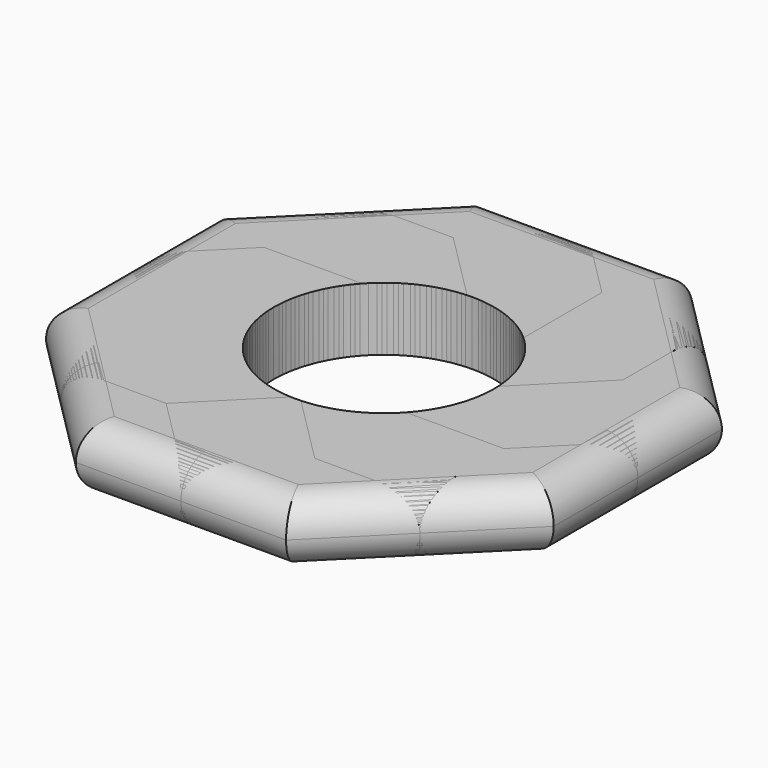
from build123d import *

# Parameters (mm, degrees)
F1_DEPTH = 3.175
F2_COUNT = 8
F3_R     = 11.049
F4_DEPTH = 12.7
F5_R     = 3.17499
F5_2_R   = 3.17499
F5_3_R   = 3.17499
F5_4_R   = 3.17499
F5_5_R   = 3.17499
F5_6_R   = 3.17499
F5_7_R   = 3.17499
F5_8_R   = 3.17499


# Not quite as in the source:
# - a fillet or chamfer is up to 0.001 mm smaller than in the source, because OpenCascade refuses the exact size


with BuildPart() as f1:
    # F0 (on Top) → F1 (new body, symmetric)
    with BuildSketch(Plane.XY):
        Polygon((5.2605122421, 0), (-5.2605122421, 0), (-12.7, -7.4394877579), (-12.7, -17.9605122421), (-5.2605122421, -25.4), (5.2605122421, -25.4), (12.7, -17.9605122421), (12.7, -7.4394877579), align=None)
    extrude(amount=F1_DEPTH, both=True)


with BuildPart() as f2_1:
    # F2: instance of F1
    add(f1.part.rotate(Axis((5.2605122421, 0, 0), (0, 0, 1)), 1 * 360 / F2_COUNT))


with BuildPart() as f2_2:
    # F2: instance of F1
    add(f1.part.rotate(Axis((5.2605122421, 0, 0), (0, 0, 1)), 2 * 360 / F2_COUNT))


with BuildPart() as f2_3:
    # F2: instance of F1
    add(f1.part.rotate(Axis((5.2605122421, 0, 0), (0, 0, 1)), 3 * 360 / F2_COUNT))


with BuildPart() as f2_4:
    # F2: instance of F1
    add(f1.part.rotate(Axis((5.2605122421, 0, 0), (0, 0, 1)), 4 * 360 / F2_COUNT))


with BuildPart() as f2_5:
    # F2: instance of F1
    add(f1.part.rotate(Axis((5.2605122421, 0, 0), (0, 0, 1)), 5 * 360 / F2_COUNT))


with BuildPart() as f2_6:
    # F2: instance of F1
    add(f1.part.rotate(Axis((5.2605122421, 0, 0), (0, 0, 1)), 6 * 360 / F2_COUNT))


with BuildPart() as f2_7:
    # F2: instance of F1
    add(f1.part.rotate(Axis((5.2605122421, 0, 0), (0, 0, 1)), 7 * 360 / F2_COUNT))


with BuildPart() as f4_tool:
    # F3 (on Top) → F4 (new body, symmetric)
    with BuildSketch(Plane.XY):
        with Locations((5.2605122421, 0)):
            Circle(F3_R)
    extrude(amount=F4_DEPTH, both=True)


with BuildPart() as f1_1:
    add(f1.part)

    # F4: cut by f4_tool
    add(f4_tool.part, mode=Mode.SUBTRACT)

    # F5#7 (radius 3.175 in the source; OpenCascade refuses exactly that, so slightly less here)
    f5_7_edges = [f1_1.edges().sort_by_distance(p)[0] for p in [
        (-8.980256, -21.680256, 3.175),
        (0, -25.4, 3.175),
        (-8.980256, -21.680256, -3.175),
        (0, -25.4, -3.175),
    ]]
    fillet(f5_7_edges, radius=F5_7_R)


with BuildPart() as f2_1_1:
    add(f2_1.part)

    # F4: cut by f4_tool
    add(f4_tool.part, mode=Mode.SUBTRACT)

    # F5#8 (radius 3.175 in the source; OpenCascade refuses exactly that, so slightly less here)
    f5_8_edges = [f2_1_1.edges().sort_by_distance(p)[0] for p in [
        (10.521024, -25.4, 3.175),
        (19.501281, -21.680256, 3.175),
        (10.521024, -25.4, -3.175),
        (19.501281, -21.680256, -3.175),
    ]]
    fillet(f5_8_edges, radius=F5_8_R)


with BuildPart() as f2_2_1:
    add(f2_2.part)

    # F4: cut by f4_tool
    add(f4_tool.part, mode=Mode.SUBTRACT)

    # F5 (radius 3.175 in the source; OpenCascade refuses exactly that, so slightly less here)
    f5_edges = [f2_2_1.edges().sort_by_distance(p)[0] for p in [
        (30.660512, -5.260512, 3.175),
        (26.940768, -14.240768, 3.175),
        (26.940768, -14.240768, -3.175),
        (30.660512, -5.260512, -3.175),
    ]]
    fillet(f5_edges, radius=F5_R)


with BuildPart() as f2_3_1:
    add(f2_3.part)

    # F4: cut by f4_tool
    add(f4_tool.part, mode=Mode.SUBTRACT)

    # F5#2 (radius 3.175 in the source; OpenCascade refuses exactly that, so slightly less here)
    f5_2_edges = [f2_3_1.edges().sort_by_distance(p)[0] for p in [
        (30.660512, 5.260512, 3.175),
        (26.940768, 14.240768, 3.175),
        (30.660512, 5.260512, -3.175),
        (26.940768, 14.240768, -3.175),
    ]]
    fillet(f5_2_edges, radius=F5_2_R)


with BuildPart() as f2_4_1:
    add(f2_4.part)

    # F4: cut by f4_tool
    add(f4_tool.part, mode=Mode.SUBTRACT)

    # F5#3 (radius 3.175 in the source; OpenCascade refuses exactly that, so slightly less here)
    f5_3_edges = [f2_4_1.edges().sort_by_distance(p)[0] for p in [
        (19.501281, 21.680256, 3.175),
        (10.521024, 25.4, 3.175),
        (19.501281, 21.680256, -3.175),
        (10.521024, 25.4, -3.175),
    ]]
    fillet(f5_3_edges, radius=F5_3_R)


with BuildPart() as f2_5_1:
    add(f2_5.part)

    # F4: cut by f4_tool
    add(f4_tool.part, mode=Mode.SUBTRACT)

    # F5#4 (radius 3.175 in the source; OpenCascade refuses exactly that, so slightly less here)
    f5_4_edges = [f2_5_1.edges().sort_by_distance(p)[0] for p in [
        (0, 25.4, 3.175),
        (-8.980256, 21.680256, 3.175),
        (0, 25.4, -3.175),
        (-8.980256, 21.680256, -3.175),
    ]]
    fillet(f5_4_edges, radius=F5_4_R)


with BuildPart() as f2_6_1:
    add(f2_6.part)

    # F4: cut by f4_tool
    add(f4_tool.part, mode=Mode.SUBTRACT)

    # F5#5 (radius 3.175 in the source; OpenCascade refuses exactly that, so slightly less here)
    f5_5_edges = [f2_6_1.edges().sort_by_distance(p)[0] for p in [
        (-16.419744, 14.240768, 3.175),
        (-20.139488, 5.260512, 3.175),
        (-16.419744, 14.240768, -3.175),
        (-20.139488, 5.260512, -3.175),
    ]]
    fillet(f5_5_edges, radius=F5_5_R)


with BuildPart() as f2_7_1:
    add(f2_7.part)

    # F4: cut by f4_tool
    add(f4_tool.part, mode=Mode.SUBTRACT)

    # F5#6 (radius 3.175 in the source; OpenCascade refuses exactly that, so slightly less here)
    f5_6_edges = [f2_7_1.edges().sort_by_distance(p)[0] for p in [
        (-20.139488, -5.260512, 3.175),
        (-16.419744, -14.240768, 3.175),
        (-20.139488, -5.260512, -3.175),
        (-16.419744, -14.240768, -3.175),
    ]]
    fillet(f5_6_edges, radius=F5_6_R)


solid = Compound([f1_1.part, f2_1_1.part, f2_2_1.part, f2_3_1.part, f2_4_1.part, f2_5_1.part, f2_6_1.part, f2_7_1.part])
